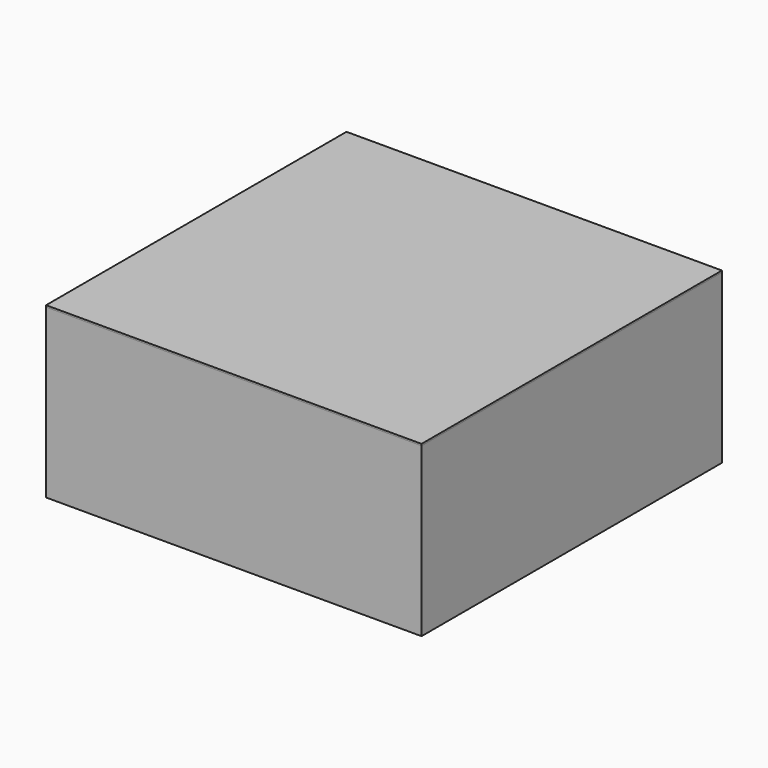
from build123d import *

# Parameters (mm, degrees)
F0_W     = 22.225
F0_H     = 9.921875
F1_DEPTH = 22.225
F2_W     = 22.225
F2_H     = 0.1016
F3_DEPTH = 22.225


# Not quite as in the source:
# - a length typed as a fraction of an inch, garbled in the dataset ("3 / 203.2 mm" for 3/8 in), is restored
# - a feature names something its author has since deleted; it is built from what else it names


with BuildPart() as f1:
    # F0 (on Front) → F1 (new body)
    with BuildSketch(Plane.XZ):
        with Locations((11.1125, 4.9609375)):
            Rectangle(F0_W, F0_H)
    extrude(amount=F1_DEPTH)


with BuildPart() as f3:
    # F2 (on Front) → F3 (new body)
    with BuildSketch(Plane.XZ):
        with Locations((11.1125, 9.972675)):
            Rectangle(F2_W, F2_H)
    extrude(amount=F3_DEPTH)


solid = Compound([f1.part, f3.part])
